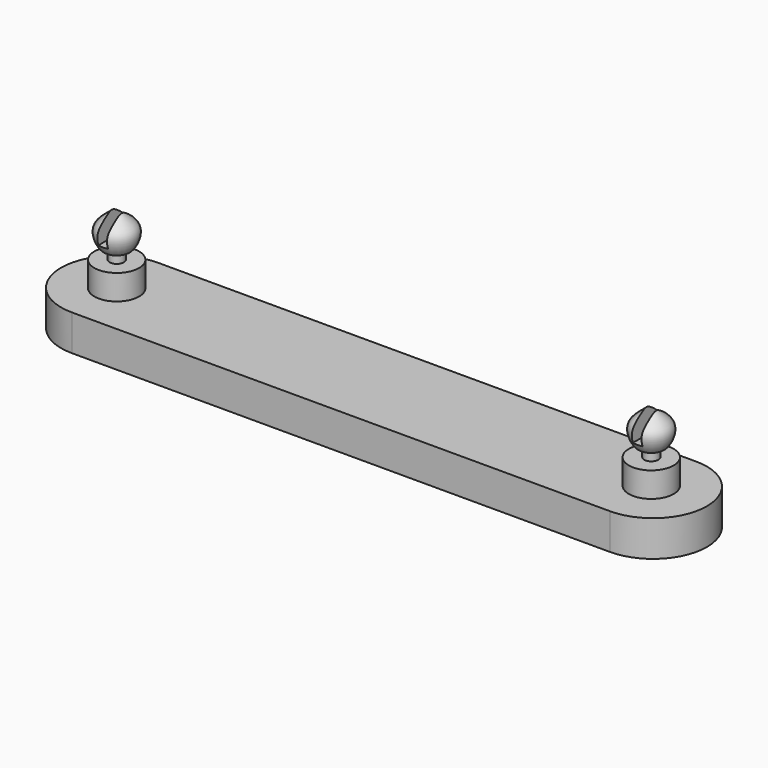
from build123d import *

# Parameters (mm, degrees)
F0_W     = 19.05
F0_H     = 7.62
F1_DEPTH = 2.54
F2_R     = 1.5875
F3_DEPTH = 1.778
F5_R     = 0.5038432106
F6_DEPTH = 2.5654
F9_DEPTH = 25.4


# Not quite as in the source:
# - a feature names something its author has since deleted; it is built from what else it names


with BuildPart() as f1:
    # F0 (on Top) → F1 (new body)
    with BuildSketch(Plane.XY):
        with Locations((-9.525, 0)):
            Rectangle(F0_W, F0_H)
        with BuildLine():
            Line((-19.05, -3.81), (-19.05, 3.81))
            ThreePointArc((-19.05, 3.81), (-22.86, 0), (-19.05, -3.81))
        make_face()
    extrude(amount=F1_DEPTH)

    # F2 (on face) → F3 (join)
    with BuildSketch(Plane.XY.offset(2.54)):
        with Locations((-18.9207902, 0)):
            Circle(F2_R)
    extrude(amount=F3_DEPTH)

    # F5 (on face) → F6 (join)
    with BuildSketch(Plane.XY.offset(4.318)):
        with Locations((-18.9207902, 0)):
            Circle(F5_R)
    extrude(amount=F6_DEPTH)

    # F4 (on Front) → F7 (revolve)
    with BuildSketch(Plane.XZ):
        with BuildLine():
            Line((-18.9207902, 7.6454), (-18.9207902, 5.4374562492))
            add(Edge.make_bspline(
                [(-18.9207902, 7.6454), (-18.7410310864, 7.4759463543), (-18.3643991229, 7.120930289), (-17.5613631578, 6.5214232415), (-17.556750871, 5.717805314), (-18.1239583371, 4.6778667739), (-18.6547230013, 5.1844366573), (-18.9207902, 5.4374562492)],
                knots=[0, 0, 0, 0, 0.1914278995, 0.4010013041, 0.591544534, 0.7954597847, 1, 1, 1, 1], degree=3))
        make_face()
    revolve(axis=Axis((-18.9207902, 0, 5.9817), (0, 0, 1)))

    # F8 (on face) → F9 (cut)
    with BuildSketch(Plane.XZ.offset(3.81)):
        Polygon((-18.5778902, 8.5426940398), (-19.2636902, 8.5426940398), (-19.2636902, 5.588), (-18.9207902, 5.588), (-18.5778902, 5.588), align=None)
    extrude(amount=-F9_DEPTH, mode=Mode.SUBTRACT)

    # F10: F1 across plane


with BuildPart() as f1_1:
    add(f1.part)
    add(f1.part.mirror(Plane.YZ))


solid = f1_1.part
